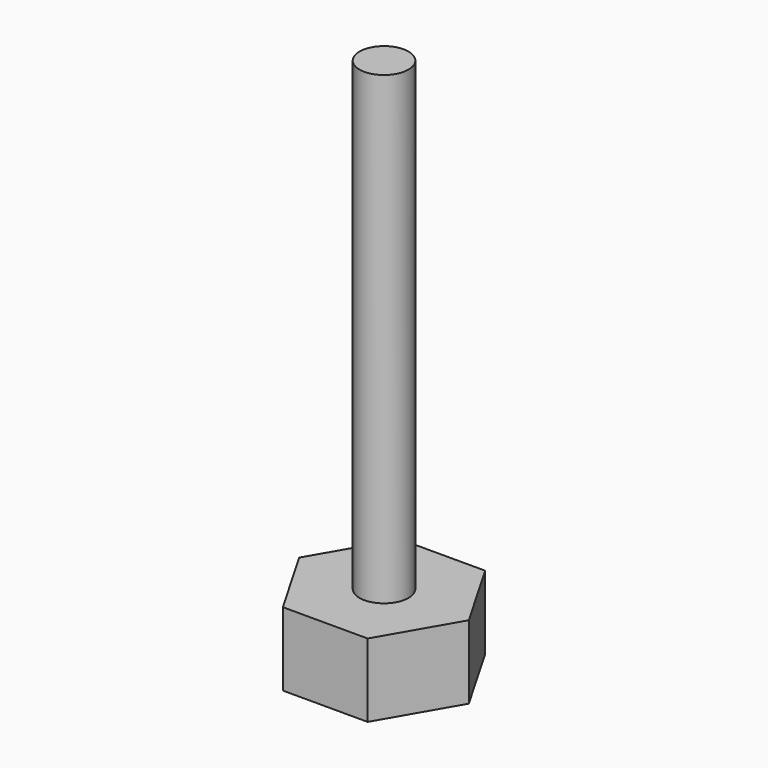
from build123d import *

# Parameters (mm, degrees)
F0_R     = 1.5875
F1_DEPTH = 4.7625
F2_DEPTH = 4.7625
F3_R     = 3.175
F4_DEPTH = 3.175
F5_R     = 1.5875
F6_DEPTH = 34.925
F8_DEPTH = 2.38125


with BuildPart() as f1:
    # F0 (on Top) → F1 (new body)
    with BuildSketch(Plane.XY):
        Polygon((2.749630657, 4.7625), (-2.749630657, 4.7625), (-5.499261314, 0), (-2.749630657, -4.7625), (2.749630657, -4.7625), (5.499261314, 0), align=None)
        Circle(F0_R, mode=Mode.SUBTRACT)
    extrude(amount=F1_DEPTH)

    # F0 (on Top) → F2 (cut)
    with BuildSketch(Plane.XY):
        Circle(F0_R)
    extrude(amount=F2_DEPTH, mode=Mode.SUBTRACT)


with BuildPart() as f4:
    # F3 (on Top) → F4 (new body)
    with BuildSketch(Plane.XY):
        Circle(F3_R)
    extrude(amount=F4_DEPTH)

    # F5 (on Top) → F6 (join)
    with BuildSketch(Plane.XY):
        Circle(F5_R)
    extrude(amount=F6_DEPTH)

    # F7 (on face) → F8 (cut)
    with BuildSketch(Plane(origin=(0, 0, 0), x_dir=(1, 0, 0), z_dir=(0, 0, -1))):
        Polygon((-0.3516971302, 1.7990323682), (-1.7338562982, 0.594937535), (-1.382159168, -1.2040948333), (0.3516971302, -1.7990323682), (1.7338562982, -0.594937535), (1.382159168, 1.2040948333), align=None)
    extrude(amount=-F8_DEPTH, mode=Mode.SUBTRACT)


solid = Compound([f1.part, f4.part])
